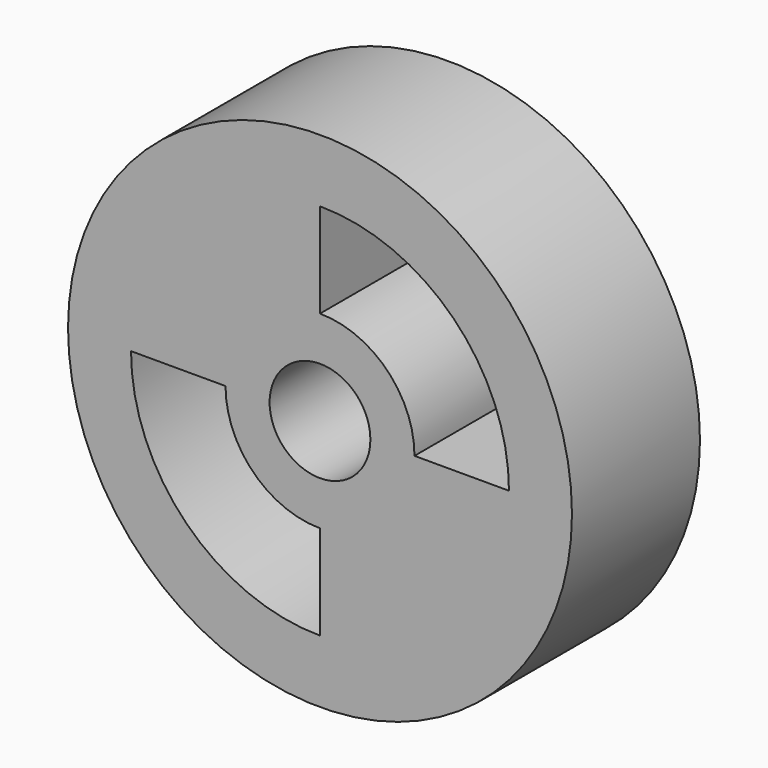
from build123d import *

# Parameters (mm, degrees)
F0_R     = 10
F0_R_2   = 2
F1_DEPTH = 6.35


# Not quite as in the source:
# - a length typed as a fraction of an inch, garbled in the dataset ("3 / 203.2 mm" for 3/8 in), is restored


with BuildPart() as f1:
    # F0 (on Front) → F1 (new body)
    with BuildSketch(Plane.XZ):
        Circle(F0_R)
        with BuildLine():
            ThreePointArc((0, 7.5), (5.3033008589, 5.3033008589), (7.5, 0))
            ThreePointArc((7.5, 0), (5.3033008589, -5.3033008589), (0, -7.5))
            ThreePointArc((0, -7.5), (-5.3033008589, -5.3033008589), (-7.5, 0))
            ThreePointArc((-7.5, 0), (-5.3033008589, 5.3033008589), (0, 7.5))
        make_face(mode=Mode.SUBTRACT)
        with BuildLine():
            ThreePointArc((0, -7.5), (5.3033008589, -5.3033008589), (7.5, 0))
            Line((7.5, 0), (3.75, 0))
            ThreePointArc((3.75, 0), (2.6516504294, -2.6516504294), (0, -3.75))
            Line((0, -3.75), (0, -7.5))
        make_face()
        with BuildLine():
            Line((0, 3.75), (0, 7.5))
            ThreePointArc((0, 7.5), (-5.3033008589, 5.3033008589), (-7.5, 0))
            Line((-7.5, 0), (-3.75, 0))
            ThreePointArc((-3.75, 0), (-2.6516504294, 2.6516504294), (0, 3.75))
        make_face()
        with BuildLine():
            ThreePointArc((0, -3.75), (2.6516504294, -2.6516504294), (3.75, 0))
            ThreePointArc((3.75, 0), (2.6516504294, 2.6516504294), (0, 3.75))
            ThreePointArc((0, 3.75), (-2.6516504294, 2.6516504294), (-3.75, 0))
            ThreePointArc((-3.75, 0), (-2.6516504294, -2.6516504294), (0, -3.75))
        make_face()
        Circle(F0_R_2, mode=Mode.SUBTRACT)
    extrude(amount=F1_DEPTH)


solid = f1.part
